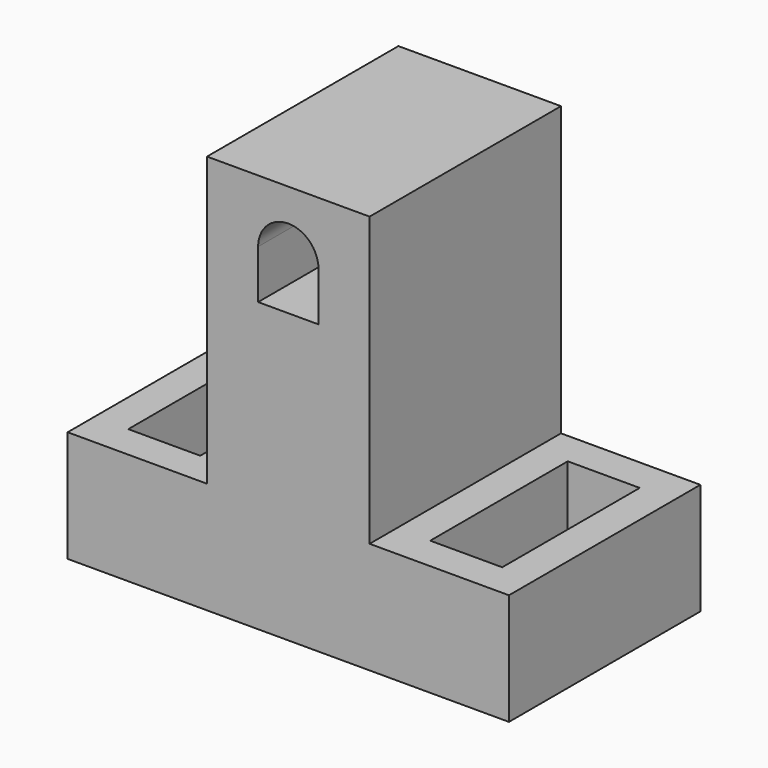
from build123d import *

# Parameters (mm, degrees)
F0_W     = 444.5
F0_H     = 654.05
F1_DEPTH = 1092.2
F2_W     = 381
F2_H     = 304.8
F3_DEPTH = 654.05
F5_DEPTH = 304.801
F7_DEPTH = 482.6


# Not quite as in the source:
# - a pattern or mirror of a feature is missing from the dataset's text; its kind, count and spacing are read off the source's solid


with BuildPart() as f1:
    # F0 (on Top) → F1 (new body)
    with BuildSketch(Plane.XY):
        Rectangle(F0_W, F0_H)
    extrude(amount=F1_DEPTH)

    # F2 (on face) → F3 (join, through all)
    with BuildSketch(Plane.XZ.offset(327.025)):
        with Locations((412.75, 152.4)):
            Rectangle(F2_W, F2_H)
        with Locations((-412.75, 152.4)):
            Rectangle(F2_W, F2_H)
    extrude(amount=-F3_DEPTH)

    # F4 (on face) → F5 (cut, through all)
    with BuildSketch(Plane.XY.offset(304.8)):
        Polygon((-314.325, -234.95), (-314.325, 168.9629166667), (-511.175, -168.9629166667), (-511.175, -234.95), align=None)
        Polygon((-511.175, -168.9629166667), (-314.325, 168.9629166667), (-314.325, 234.95), (-511.175, 234.95), align=None)
    f5 = extrude(amount=-F5_DEPTH, mode=Mode.SUBTRACT)

    # F5_copies: F5 across plane
    add(f5.mirror(Plane(origin=(0, 0, 0), x_dir=(0, 0, 1), z_dir=(1, 0, 0))), mode=Mode.SUBTRACT)

    # F6 (on face) → F7 (cut)
    with BuildSketch(Plane.XZ.offset(327.025)):
        with BuildLine():
            ThreePointArc((82.55, 920.75), (58.3716647869, 979.121664787), (0, 1003.3))
            Line((0, 1003.3), (0, 920.75))
            Line((0, 920.75), (82.55, 920.75))
        make_face()
        with BuildLine():
            Line((0, 920.75), (0, 1003.3))
            ThreePointArc((0, 1003.3), (-58.371664787, 979.1216647869), (-82.55, 920.75))
            Line((-82.55, 920.75), (0, 920.75))
        make_face()
        with BuildLine():
            Line((82.55, 920.75), (0, 920.75))
            Line((0, 920.75), (0, 838.2))
            ThreePointArc((0, 838.2), (58.3716647869, 862.378335213), (82.55, 920.75))
        make_face()
        with BuildLine():
            Line((0, 838.2), (0, 920.75))
            Line((0, 920.75), (-82.55, 920.75))
            ThreePointArc((-82.55, 920.75), (-58.371664787, 862.3783352131), (0, 838.2))
        make_face()
        with BuildLine():
            Line((82.55, 787.4), (82.55, 920.75))
            ThreePointArc((82.55, 920.75), (58.3716647869, 862.378335213), (0, 838.2))
            Line((0, 838.2), (0, 787.4))
            Line((0, 787.4), (82.55, 787.4))
        make_face()
        with BuildLine():
            ThreePointArc((0, 838.2), (-58.371664787, 862.3783352131), (-82.55, 920.75))
            Line((-82.55, 920.75), (-82.55, 787.4))
            Line((-82.55, 787.4), (0, 787.4))
            Line((0, 787.4), (0, 838.2))
        make_face()
    extrude(amount=-F7_DEPTH, mode=Mode.SUBTRACT)


solid = f1.part
